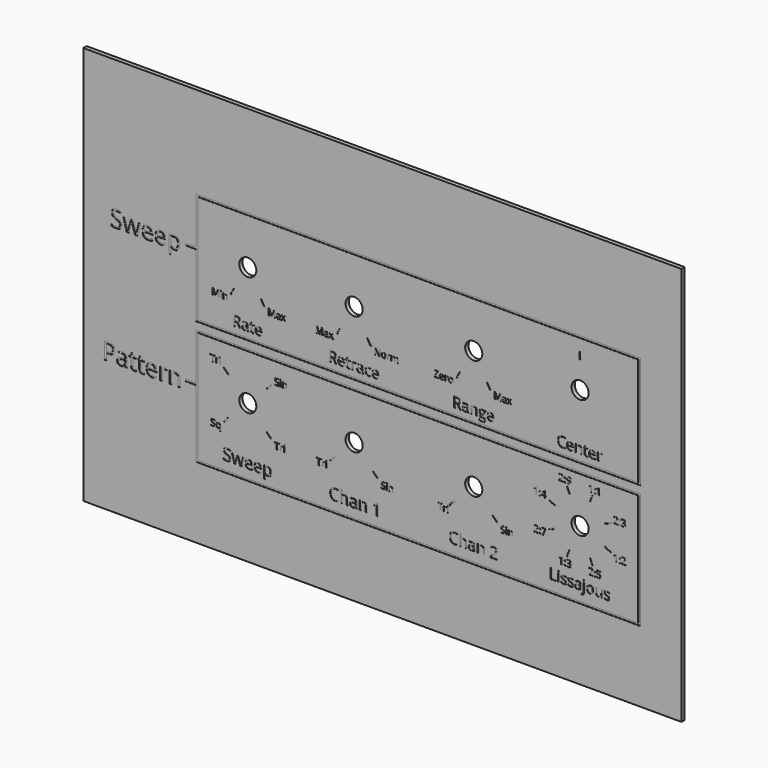
from build123d import *

# Parameters (mm, degrees)
F0_W           = 228.6
F0_H           = 152.4
F1_DEPTH       = 1.5748
F3_D           = 6.5278
F4_TEXT_SIZE   = 6.2033173909
F4_TEXT_SIZE_2 = 6.1684796357
F4_TEXT_SIZE_3 = 5.8483234998
F4_TEXT_SIZE_4 = 5.5386111111
F4_TEXT_SIZE_5 = 8.8194444444
F5_DEPTH       = 0.127
F6_W           = 0.381
F6_H           = 2.54
F6_TEXT_SIZE   = 3.5277777778
F7_DEPTH       = 0.127
F8_W           = 168.275
F8_H           = 41.275
F8_W_2         = 3.96875
F8_H_2         = 0.79375
F8_H_3         = 42.8625
F9_DEPTH       = 0.127


# Not quite as in the source:
# - Text() gives the source's letters only with a copy of the font that has no kerning and outlines rounded to 1/6400 em; it was checked with that copy


with BuildPart() as f1:
    # F0 (on Front) → F1 (new body)
    with BuildSketch(Plane.XZ):
        Rectangle(F0_W, F0_H)
    extrude(amount=F1_DEPTH)

    # F3 (through all)
    with Locations(Plane.XZ.offset(1.5748)):
        with Locations((-51.435, 22.86), (-10.795, 22.86), (34.925, 22.86), (75.565, 22.86), (75.565, -22.86), (34.925, -22.86), (-10.795, -22.86), (-51.435, -22.86)):
            Hole(F3_D / 2)

    # F4 (on face) → F5 (cut)
    with BuildSketch(Plane.XZ.offset(1.5748)):
        with Locations((-60.96, -44.8777885214)):
            Text('Sweep', F4_TEXT_SIZE, font='Open Sans', text_align=(TextAlign.LEFT, TextAlign.BOTTOM))
        with Locations((-20.32, -44.8527053377)):
            Text('Chan 1', F4_TEXT_SIZE_2, font='Open Sans', text_align=(TextAlign.LEFT, TextAlign.BOTTOM))
        with Locations((25.4, -44.6221929198)):
            Text('Chan 2', F4_TEXT_SIZE_3, font='Open Sans', text_align=(TextAlign.LEFT, TextAlign.BOTTOM))
        with Locations((63.7984803168, -44.3992)):
            Text('Lissajous', F4_TEXT_SIZE_4, font='Open Sans', text_align=(TextAlign.LEFT, TextAlign.BOTTOM))
        with Locations((-20.6156498264, 1.3208)):
            Text('Retrace', F4_TEXT_SIZE_4, font='Open Sans', text_align=(TextAlign.LEFT, TextAlign.BOTTOM))
        with Locations((26.8680516493, 1.3208)):
            Text('Range', F4_TEXT_SIZE_4, font='Open Sans', text_align=(TextAlign.LEFT, TextAlign.BOTTOM))
        with Locations((66.7620699653, 1.3208)):
            Text('Center', F4_TEXT_SIZE_4, font='Open Sans', text_align=(TextAlign.LEFT, TextAlign.BOTTOM))
        with Locations((-57.2527051866, 1.3208)):
            Text('Rate', F4_TEXT_SIZE_4, font='Open Sans', text_align=(TextAlign.LEFT, TextAlign.BOTTOM))
        with Locations((-103.9189626736, 19.685)):
            Text('Sweep', F4_TEXT_SIZE_5, font='Open Sans', text_align=(TextAlign.LEFT, TextAlign.BOTTOM))
        with Locations((-107.0994748264, -26.035)):
            Text('Pattern', F4_TEXT_SIZE_5, font='Open Sans', text_align=(TextAlign.LEFT, TextAlign.BOTTOM))
    extrude(amount=-F5_DEPTH, mode=Mode.SUBTRACT)

    # F6 (on face) → F7 (cut)
    with BuildSketch(Plane.XZ.offset(1.5748)):
        Polygon((-42.2090303616, -31.8165619547), (-44.0050815859, -30.0205107305), (-44.2744892695, -30.2899184141), (-42.4784380453, -32.0859696384), align=None)
        Polygon((-42.2090303616, -13.9034380453), (-42.4784380453, -13.6340303616), (-44.2744892695, -15.4300815859), (-44.0050815859, -15.6994892695), align=None)
        Polygon((80.3091585435, -10.9087876125), (79.3371426253, -13.2554416251), (79.6891407272, -13.4012440128), (80.6611566454, -11.0545900003), align=None)
        Polygon((85.0237559872, -18.7358592728), (85.1695583749, -19.0878573747), (87.5162123875, -18.1158414565), (87.3704099997, -17.7638433546), align=None)
        Polygon((85.1695583749, -26.6321426253), (85.0237559872, -26.9841407272), (87.3704099997, -27.9561566454), (87.5162123875, -27.6041585435), align=None)
        Polygon((79.6891407272, -32.3187559872), (79.3371426253, -32.4645583749), (80.3091585435, -34.8112123875), (80.6611566454, -34.6654099997), align=None)
        Polygon((71.7928573747, -32.4645583749), (71.4408592728, -32.3187559872), (70.4688433546, -34.6654099997), (70.8208414565, -34.8112123875), align=None)
        Polygon((66.1062440128, -26.9841407272), (65.9604416251, -26.6321426253), (63.6137876125, -27.6041585435), (63.7595900003, -27.9561566454), align=None)
        Polygon((65.9604416251, -19.0878573747), (66.1062440128, -18.7358592728), (63.7595900003, -17.7638433546), (63.6137876125, -18.1158414565), align=None)
        Polygon((71.4408592728, -13.4012440128), (71.7928573747, -13.2554416251), (70.8208414565, -10.9087876125), (70.4688433546, -11.0545900003), align=None)
        Polygon((27.4950815859, -30.0205107305), (25.6990303616, -31.8165619547), (25.9684380453, -32.0859696384), (27.7644892695, -30.2899184141), align=None)
        Polygon((44.1509696384, -31.8165619547), (42.3549184141, -30.0205107305), (42.0855107305, -30.2899184141), (43.8815619547, -32.0859696384), align=None)
        Polygon((-18.2249184141, -30.0205107305), (-20.0209696384, -31.8165619547), (-19.7515619547, -32.0859696384), (-17.9555107305, -30.2899184141), align=None)
        Polygon((-1.5690303616, -31.8165619547), (-3.3650815859, -30.0205107305), (-3.6344892695, -30.2899184141), (-1.8384380453, -32.0859696384), align=None)
        Polygon((-58.8649184141, -30.0205107305), (-60.6609696384, -31.8165619547), (-60.3915619547, -32.0859696384), (-58.5955107305, -30.2899184141), align=None)
        Polygon((-16.1184735337, 14.0204733668), (-17.3884735337, 11.8207688412), (-17.0585178549, 11.6302688412), (-15.7885178549, 13.8299733668), align=None)
        Polygon((-4.2015264663, 11.8207688412), (-5.4715264663, 14.0204733668), (-5.8014821451, 13.8299733668), (-4.5314821451, 11.6302688412), align=None)
        Polygon((-56.7584735337, 14.0204733668), (-58.0284735337, 11.8207688412), (-57.6985178549, 11.6302688412), (-56.4285178549, 13.8299733668), align=None)
        Polygon((-44.8415264663, 11.8207688412), (-46.1115264663, 14.0204733668), (-46.4414821451, 13.8299733668), (-45.1714821451, 11.6302688412), align=None)
        with Locations((75.565, 34.4469913886)):
            Rectangle(F6_W, F6_H)
        Polygon((40.2484735337, 14.0204733668), (40.0834956943, 13.9252233668), (41.3534956943, 11.7255188412), (41.5184735337, 11.8207688412), align=None)
        Polygon((41.3534956943, 11.7255188412), (40.0834956943, 13.9252233668), (39.9185178549, 13.8299733668), (41.1885178549, 11.6302688412), align=None)
        Polygon((29.6015264663, 14.0204733668), (28.3315264663, 11.8207688412), (28.6614821451, 11.6302688412), (29.9314821451, 13.8299733668), align=None)
        Polygon((-58.5955107305, -15.4300815859), (-60.3915619547, -13.6340303616), (-60.6609696384, -13.9034380453), (-58.8649184141, -15.6994892695), align=None)
        with Locations((-41.275, -34.925)):
            Text('Tri', F6_TEXT_SIZE, font='Open Sans', text_align=(TextAlign.LEFT, TextAlign.BOTTOM))
        with Locations((78.74, -38.1)):
            Text('2:5', F6_TEXT_SIZE, font='Open Sans', text_align=(TextAlign.LEFT, TextAlign.BOTTOM))
        with Locations((67.3954383681, -38.1)):
            Text('1:3', F6_TEXT_SIZE, font='Open Sans', text_align=(TextAlign.LEFT, TextAlign.BOTTOM))
        with Locations((57.8428776042, -30.48)):
            Text('2:7', F6_TEXT_SIZE, font='Open Sans', text_align=(TextAlign.LEFT, TextAlign.BOTTOM))
        with Locations((57.7342881944, -17.78)):
            Text('1:4', F6_TEXT_SIZE, font='Open Sans', text_align=(TextAlign.LEFT, TextAlign.BOTTOM))
        with Locations((67.3777994792, -10.16)):
            Text('2:9', F6_TEXT_SIZE, font='Open Sans', text_align=(TextAlign.LEFT, TextAlign.BOTTOM))
        with Locations((78.74, -10.16)):
            Text('1:1', F6_TEXT_SIZE, font='Open Sans', text_align=(TextAlign.LEFT, TextAlign.BOTTOM))
        with Locations((88.265, -17.78)):
            Text('2:3', F6_TEXT_SIZE, font='Open Sans', text_align=(TextAlign.LEFT, TextAlign.BOTTOM))
        with Locations((88.265, -30.48)):
            Text('1:2', F6_TEXT_SIZE, font='Open Sans', text_align=(TextAlign.LEFT, TextAlign.BOTTOM))
        with Locations((-41.275, -13.335)):
            Text('Sin', F6_TEXT_SIZE, font='Open Sans', text_align=(TextAlign.LEFT, TextAlign.BOTTOM))
        with Locations((-65.6188715278, -34.925)):
            Text('Sq', F6_TEXT_SIZE, font='Open Sans', text_align=(TextAlign.LEFT, TextAlign.BOTTOM))
        with Locations((-25.1927430556, -34.925)):
            Text('Tri', F6_TEXT_SIZE, font='Open Sans', text_align=(TextAlign.LEFT, TextAlign.BOTTOM))
        with Locations((-0.635, -34.925)):
            Text('Sin', F6_TEXT_SIZE, font='Open Sans', text_align=(TextAlign.LEFT, TextAlign.BOTTOM))
        with Locations((45.085, -34.925)):
            Text('Sin', F6_TEXT_SIZE, font='Open Sans', text_align=(TextAlign.LEFT, TextAlign.BOTTOM))
        with Locations((21.1622569444, -34.925)):
            Text('Tri', F6_TEXT_SIZE, font='Open Sans', text_align=(TextAlign.LEFT, TextAlign.BOTTOM))
        with Locations((-3.175, 9.2075)):
            Text('Norm', F6_TEXT_SIZE, font='Open Sans', text_align=(TextAlign.LEFT, TextAlign.BOTTOM))
        with Locations((-25.5681206597, 9.2075)):
            Text('Max', F6_TEXT_SIZE, font='Open Sans', text_align=(TextAlign.LEFT, TextAlign.BOTTOM))
        with Locations((-65.2423914931, 9.2075)):
            Text('Min', F6_TEXT_SIZE, font='Open Sans', text_align=(TextAlign.LEFT, TextAlign.BOTTOM))
        with Locations((-43.815, 9.2075)):
            Text('Max', F6_TEXT_SIZE, font='Open Sans', text_align=(TextAlign.LEFT, TextAlign.BOTTOM))
        with Locations((42.545, 9.2075)):
            Text('Max', F6_TEXT_SIZE, font='Open Sans', text_align=(TextAlign.LEFT, TextAlign.BOTTOM))
        with Locations((19.7103559028, 9.2075)):
            Text('Zero', F6_TEXT_SIZE, font='Open Sans', text_align=(TextAlign.LEFT, TextAlign.BOTTOM))
        with Locations((-65.8327430556, -13.335)):
            Text('Tri', F6_TEXT_SIZE, font='Open Sans', text_align=(TextAlign.LEFT, TextAlign.BOTTOM))
    extrude(amount=-F7_DEPTH, mode=Mode.SUBTRACT)

    # F8 (on face) → F9 (cut)
    with BuildSketch(Plane.XZ.offset(1.5748)):
        Polygon((98.58375, 41.11625), (-71.27875, 41.11625), (-71.27875, 23.256875), (-71.27875, 22.463125), (-71.27875, -1.74625), (98.58375, -1.74625), align=None)
        with Locations((13.6525, 19.685)):
            Rectangle(F8_W, F8_H, mode=Mode.SUBTRACT)
        with Locations((-73.263125, 22.86)):
            Rectangle(F8_W_2, F8_H_2)
        Polygon((98.58375, -4.60375), (-71.27875, -4.60375), (-71.27875, -22.463125), (-71.27875, -23.256875), (-71.27875, -49.05375), (98.58375, -49.05375), align=None)
        with Locations((13.6525, -26.82875)):
            Rectangle(F8_W, F8_H_3, mode=Mode.SUBTRACT)
        with Locations((-73.263125, -22.86)):
            Rectangle(F8_W_2, F8_H_2)
    extrude(amount=-F9_DEPTH, mode=Mode.SUBTRACT)


solid = f1.part
